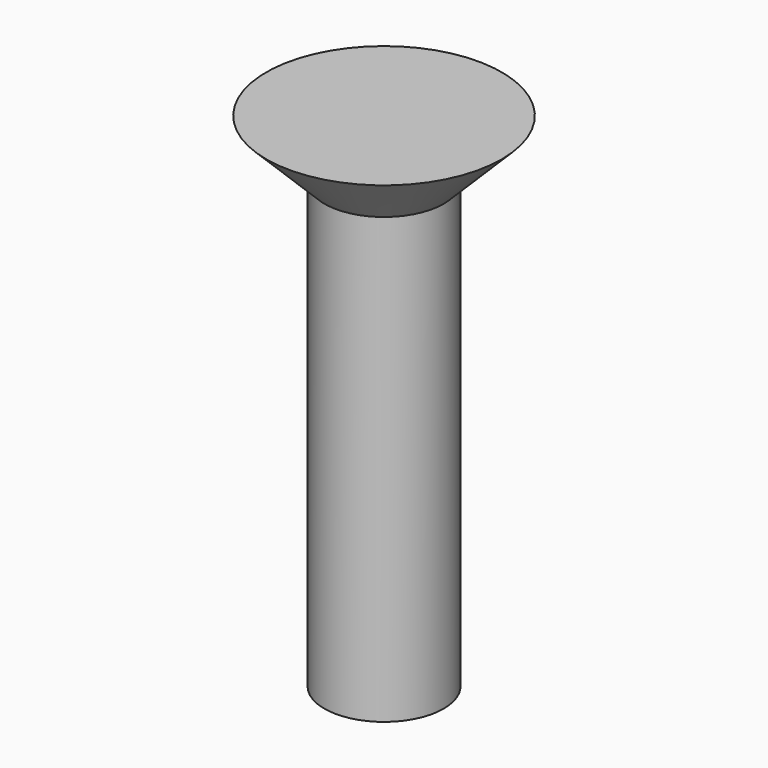
from build123d import *

# Parameters (mm, degrees)
F0_R        = 3.75
F1_DEPTH    = 2
F2_R        = 1.9
F3_DEPTH    = 14
F4_S5_R     = 1.9
F4_T6_DEPTH = 7


# Not quite as in the source:
# - a fillet or chamfer that OpenCascade refuses, or shapes differently, is made with other operations: its cross-section is extruded or revolved along the edge and cut away or added


with BuildPart() as f1:
    # F0 (on Top) → F1 (new body)
    with BuildSketch(Plane.XY):
        Circle(F0_R)
    extrude(amount=F1_DEPTH)

    # F2 (on face) → F3 (join)
    with BuildSketch(Plane(origin=(0, 0, 0), x_dir=(1, 0, 0), z_dir=(0, 0, -1))):
        Circle(F2_R)
    extrude(amount=F3_DEPTH)

    # F4: chamfer of 2 on 1 edges, made by hand


with BuildPart() as f4_tool2:
    # F4_s3 → F4_t4 (revolve)
    with BuildSketch(Plane.XZ):
        Polygon((3.75, 2), (1.75, 0), (3.75, 0), align=None)
    revolve(axis=Axis((0, 0, 0), (0, 0, 1)))

    # F4_s5 → F4_t6 (cut, symmetric)
    with BuildSketch(Plane.XY.offset(1)):
        Circle(F4_S5_R)
    extrude(amount=F4_T6_DEPTH, both=True, mode=Mode.SUBTRACT)


with BuildPart() as f1_1:
    add(f1.part)

    # F4_t1: cut F4_tool2
    add(f4_tool2.part, mode=Mode.SUBTRACT)


solid = f1_1.part
